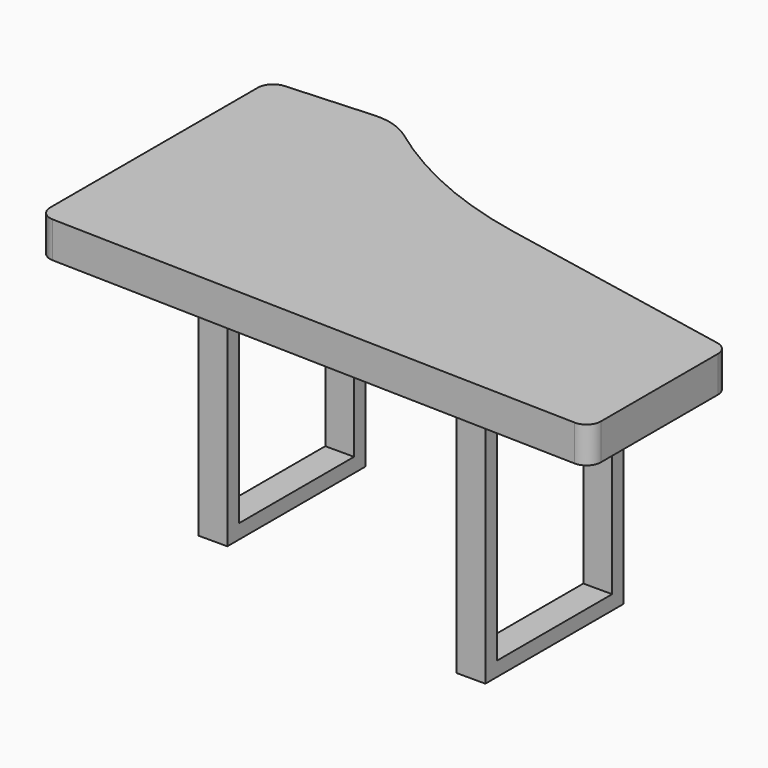
from build123d import *

# Parameters (mm, degrees)
F1_DEPTH    = 63.5
F3_T1_DEPTH = 63.5
F2_W        = 50.8
F2_H        = 304.8
F4_DEPTH    = 3.175
F7_W        = 50.8
F7_H        = 25.4
F7_W_2      = 44.45
F7_H_2      = 19.05
F11_W       = 50.8
F11_H       = 25.4
F13_R       = 103.4882786099
F14_R       = 27.1342571694
F15_R       = 25.4


# Not quite as in the source:
# - a fillet or chamfer that OpenCascade refuses, or shapes differently, is made with other operations: its cross-section is extruded or revolved along the edge and cut away or added


with BuildPart() as f1:
    # F0 (on Top) → F1 (new body)
    with BuildSketch(Plane.XY):
        Polygon((-990.6, 25.4), (0, 0), (0, 304.8), (-678.6715388298, 438.15), (-774.7, 546.1), (-990.6, 533.4), align=None)
    extrude(amount=F1_DEPTH)

    # F3: fillet of radius 736.2487387041 on 1 edges, made by hand

    # F3_s2 → F3_t1 (join)
    with BuildSketch(Plane.XY):
        with BuildLine():
            ThreePointArc((-450.1285521095, 393.2443195118), (-621.8672665328, 449.5998222637), (-774.7, 546.1))
            Line((-774.7, 546.1), (-678.6715388298, 438.15))
            Line((-678.6715388298, 438.15), (-450.1285521095, 393.2443195118))
        make_face()
    extrude(amount=F3_T1_DEPTH)

    # F13
    f13_edges = [f1.edges().sort_by_distance(p)[0] for p in [
        (-774.7, 546.1, 31.75),
    ]]
    fillet(f13_edges, radius=F13_R)

    # F14
    f14_edges = [f1.edges().sort_by_distance(p)[0] for p in [
        (-990.6, 533.4, 31.75),
    ]]
    fillet(f14_edges, radius=F14_R)

    # F15
    f15_edges = [f1.edges().sort_by_distance(p)[0] for p in [
        (-990.6, 25.4, 31.75),
        (0, 0, 31.75),
        (0, 304.8, 31.75),
    ]]
    fillet(f15_edges, radius=F15_R)


with BuildPart() as f4:
    # F2 (on face) → F4 (new body)
    with BuildSketch(Plane(origin=(0, 0, 0), x_dir=(1, 0, 0), z_dir=(0, 0, -1))):
        with Locations((-228.6, -177.7892106534)):
            Rectangle(F2_W, F2_H)
    extrude(amount=F4_DEPTH)


with BuildPart() as f4b:
    # F2 (on face) → F4, piece 2 (new body)
    with BuildSketch(Plane(origin=(0, 0, 0), x_dir=(1, 0, 0), z_dir=(0, 0, -1))):
        with Locations((-762, -275.6809043643)):
            Rectangle(F2_W, F2_H)
    extrude(amount=F4_DEPTH)


with BuildPart() as f8:
    # F8: sweep along a path in F5
    with BuildLine(Plane(origin=(-787.4, 0, 0), x_dir=(0, -1, 0), z_dir=(-1, 0, 0))) as f8_path:
        Line((-199.4809043643, -3.175), (-123.2809043643, -3.175))
        Line((-123.2809043643, -3.175), (-123.2809043643, -409.575))
        Line((-123.2809043643, -409.575), (-428.0809043643, -409.575))
        Line((-428.0809043643, -409.575), (-428.0809043643, -3.175))
        Line((-428.0809043643, -3.175), (-351.8809043643, -3.175))
    # F7 (on line) → F8 (sweep)
    with BuildSketch(Plane.XZ.offset(-351.8809043643)):
        with Locations((-762, -15.875)):
            Rectangle(F7_W, F7_H)
        with Locations((-762, -15.875)):
            Rectangle(F7_W_2, F7_H_2, mode=Mode.SUBTRACT)
    sweep(path=f8_path.line, transition=Transition.RIGHT)


with BuildPart() as f12:
    # F12: sweep along a path in F9
    with BuildLine(Plane.YZ.offset(-203.2)) as f12_path:
        Line((88.8892106534, -3.175), (25.3892106534, -3.175))
        Line((25.3892106534, -3.175), (25.3892106534, -409.575))
        Line((25.3892106534, -409.575), (330.1892106534, -409.575))
        Line((330.1892106534, -409.575), (330.1892106534, -3.175))
        Line((330.1892106534, -3.175), (266.6892106534, -3.175))
    # F11 (on line) → F12 (sweep)
    with BuildSketch(Plane.XZ.offset(-88.8892106534)):
        with Locations((-228.6, -15.875)):
            Rectangle(F11_W, F11_H)
    sweep(path=f12_path.line, transition=Transition.RIGHT)


solid = Compound([f1.part, f4.part, f4b.part, f8.part, f12.part])
